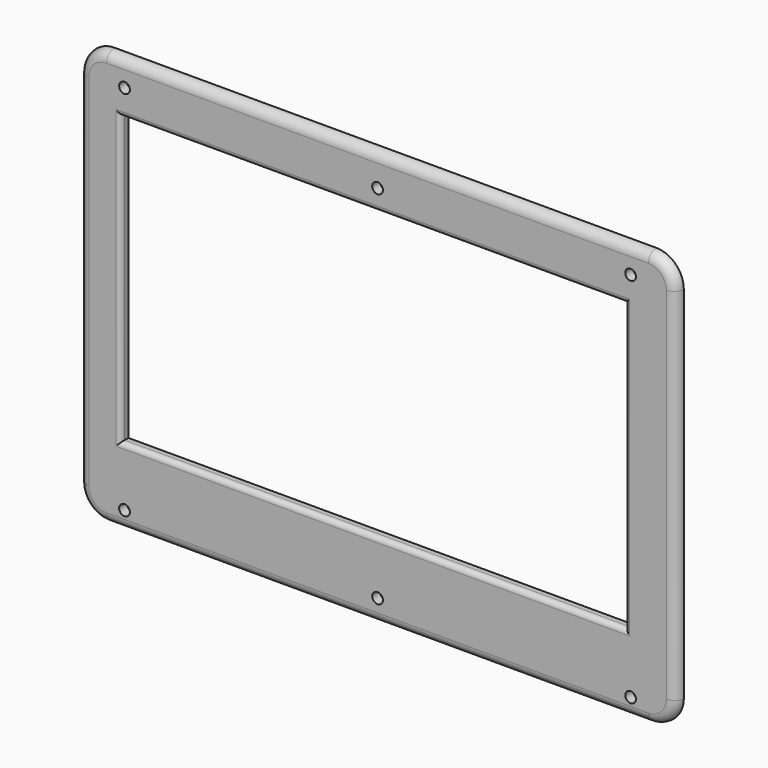
from build123d import *

# Parameters (mm, degrees)
F0_R     = 1.65
F0_W     = 155.4
F0_H     = 88.4
F1_DEPTH = 3
F2_R     = 2.99999
F3_R     = 1.5


# Not quite as in the source:
# - a fillet or chamfer is up to 0.001 mm smaller than in the source, because OpenCascade refuses the exact size


with BuildPart() as f1:
    # F0 (on Front) → F1 (new body)
    with BuildSketch(Plane.XZ):
        with BuildLine():
            Line((83.5, 64), (-83.5, 64))
            ThreePointArc((-83.5, 64), (-89.5104076401, 61.5104076401), (-92, 55.5))
            Line((-92, 55.5), (-92, -55.5))
            ThreePointArc((-92, -55.5), (-89.5104076401, -61.5104076401), (-83.5, -64))
            Line((-83.5, -64), (83.5, -64))
            ThreePointArc((83.5, -64), (89.5104076401, -61.5104076401), (92, -55.5))
            Line((92, -55.5), (92, 55.5))
            ThreePointArc((92, 55.5), (89.5104076401, 61.5104076401), (83.5, 64))
        make_face()
        with Locations((-78, -58.5)):
            Circle(F0_R, mode=Mode.SUBTRACT)
        with Locations((0, -57)):
            Circle(F0_R, mode=Mode.SUBTRACT)
        with Locations((78, -58.5)):
            Circle(F0_R, mode=Mode.SUBTRACT)
        with BuildLine():
            Line((-83.5, -50.5), (-83.5, 52.5))
            Line((-83.5, 52.5), (83.5, 52.5))
            Line((83.5, 52.5), (83.5, -51.5))
            ThreePointArc((83.5, -51.5), (83.2071067812, -52.2071067812), (82.5, -52.5))
            Line((82.5, -52.5), (47.5, -52.5))
            ThreePointArc((47.5, -52.5), (46.7928932188, -52.2071067812), (46.5, -51.5))
            ThreePointArc((46.5, -51.5), (46.2071067812, -50.7928932188), (45.5, -50.5))
            Line((45.5, -50.5), (-83.5, -50.5))
        make_face(mode=Mode.SUBTRACT)
        with Locations((-78, 56.1)):
            Circle(F0_R, mode=Mode.SUBTRACT)
        with Locations((0, 54.25)):
            Circle(F0_R, mode=Mode.SUBTRACT)
        with Locations((78, 56.1)):
            Circle(F0_R, mode=Mode.SUBTRACT)
        with BuildLine():
            Line((83.5, 52.5), (-83.5, 52.5))
            Line((-83.5, 52.5), (-83.5, -50.5))
            Line((-83.5, -50.5), (45.5, -50.5))
            ThreePointArc((45.5, -50.5), (46.2071067812, -50.7928932188), (46.5, -51.5))
            ThreePointArc((46.5, -51.5), (46.7928932188, -52.2071067812), (47.5, -52.5))
            Line((47.5, -52.5), (82.5, -52.5))
            ThreePointArc((82.5, -52.5), (83.2071067812, -52.2071067812), (83.5, -51.5))
            Line((83.5, -51.5), (83.5, 52.5))
        make_face()
        with Locations((-1.5, 3.7)):
            Rectangle(F0_W, F0_H, mode=Mode.SUBTRACT)
    extrude(amount=F1_DEPTH)

    # F2 (radius 3 in the source; OpenCascade refuses exactly that, so slightly less here)
    f2_edges = [f1.edges().sort_by_distance(p)[0] for p in [
        (92, -3, 0),
    ]]
    fillet(f2_edges, radius=F2_R)

    # F3
    f3_edges = [f1.edges().sort_by_distance(p)[0] for p in [
        (-79.2, -3, 3.7),
        (-1.5, -3, 47.9),
        (76.2, -3, 3.7),
        (-1.5, -3, -40.5),
    ]]
    fillet(f3_edges, radius=F3_R)


solid = f1.part
